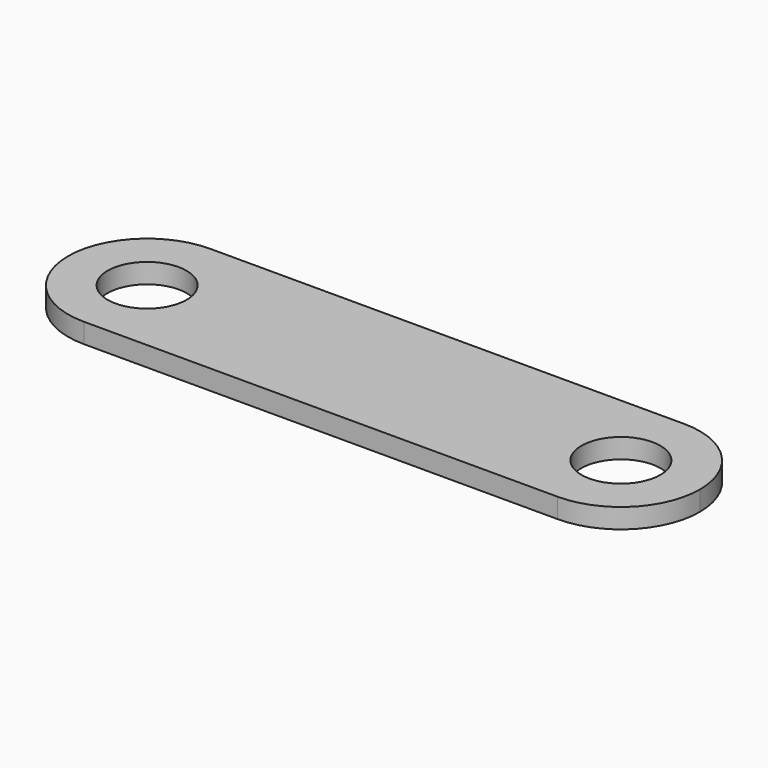
from build123d import *

# Parameters (mm, degrees)
F0_W     = 101.6
F0_H     = 25.4
F0_R     = 6.35
F1_DEPTH = 3.175
F2_R     = 12.69999


# Not quite as in the source:
# - a fillet or chamfer is up to 0.001 mm smaller than in the source, because OpenCascade refuses the exact size


with BuildPart() as f1:
    # F0 (on Top) → F1 (new body)
    with BuildSketch(Plane.XY):
        Rectangle(F0_W, F0_H)
        with Locations((-38.1, 0)):
            Circle(F0_R, mode=Mode.SUBTRACT)
        with Locations((38.1, 0)):
            Circle(F0_R, mode=Mode.SUBTRACT)
    extrude(amount=F1_DEPTH)

    # F2 (radius 12.7 in the source; OpenCascade refuses exactly that, so slightly less here)
    f2_edges = [f1.edges().sort_by_distance(p)[0] for p in [
        (-50.8, -12.7, 1.5875),
        (50.8, -12.7, 1.5875),
        (-50.8, 12.7, 1.5875),
        (50.8, 12.7, 1.5875),
    ]]
    fillet(f2_edges, radius=F2_R)


solid = f1.part
